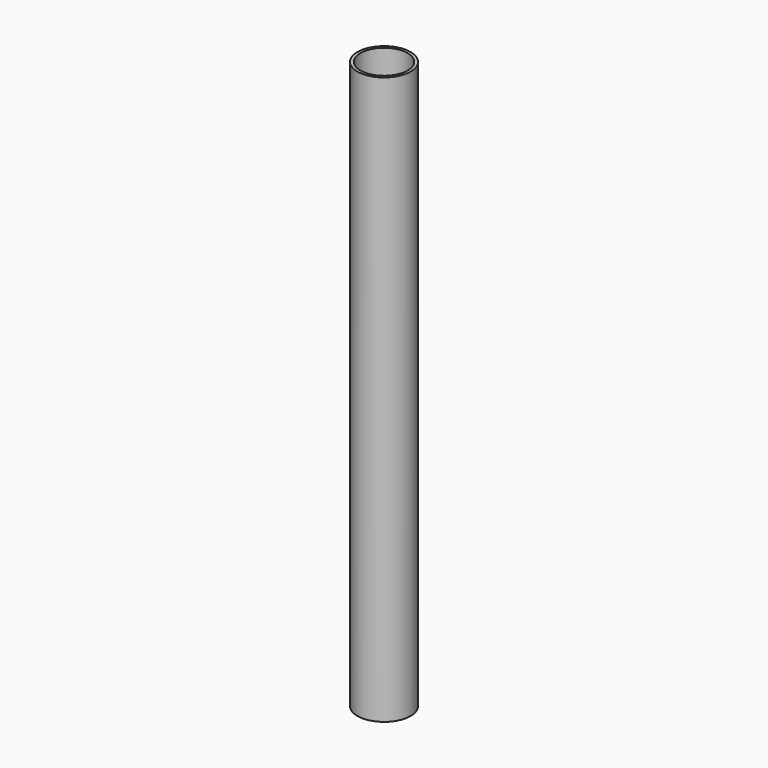
from build123d import *

# Parameters (mm, degrees)
F0_R     = 14.2875
F0_R_2   = 12.7
F1_DEPTH = 304.8


# Not quite as in the source:
# - a feature names something its author has since deleted; it is built from what else it names


with BuildPart() as f1:
    # F0 (on Top) → F1 (new body)
    with BuildSketch(Plane.XY):
        Circle(F0_R)
        Circle(F0_R_2, mode=Mode.SUBTRACT)
    extrude(amount=F1_DEPTH)


solid = f1.part
